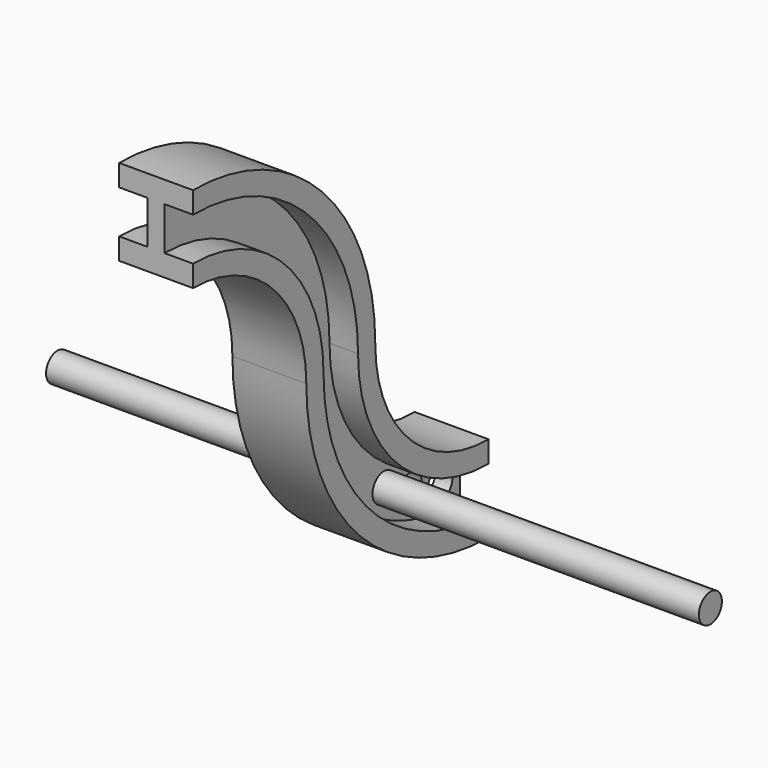
from build123d import *

# Parameters (mm, degrees)
F3_R     = 29.6946462183
F4_DEPTH = 673.1
F5_R     = 31.777125294
F5_R_2   = 32.6810684337
F6_DEPTH = 673.101


# Not quite as in the source:
# - a feature of the source that left no trace in its solid (it failed there, or was rolled back) is left out


with BuildPart() as f2:
    # F2: sweep along a path in F1
    with BuildLine(Plane.YZ) as f2_path:
        ThreePointArc((0, 0), (269.4076836321, -111.5923163679), (381, -381))
        ThreePointArc((381, -381), (492.5923163679, -650.4076836321), (762, -762))
    # F0 (on Front) → F2 (sweep)
    with BuildSketch(Plane.XZ):
        Polygon((76.2, 88.9), (0, 88.9), (-76.2, 88.9), (-76.2, 44.45), (-17.3748321831, 44.45), (-17.3748321831, 0), (-17.3748321831, -44.45), (-76.2, -44.45), (-76.2, -88.9), (0, -88.9), (76.2, -88.9), (76.2, -44.45), (17.3748321831, -44.45), (17.3748321831, 0), (17.3748321831, 44.45), (76.2, 44.45), align=None)
    sweep(path=f2_path.line)

    # F3 (on face) → F4 (join, symmetric)
    with BuildSketch(Plane.YZ.offset(17.3748321831)):
        with Locations((565.865278244, -699.9046206474)):
            Circle(F3_R)
    extrude(amount=F4_DEPTH, both=True)

    # F5 (on face) → F6 (cut, through all)
    with BuildSketch(Plane.YZ.offset(17.3748321831)):
        with Locations((631.9480538368, -732.2566509247)):
            Circle(F5_R)
        with Locations((709.6602916718, -753.0537247658)):
            Circle(F5_R_2)
    extrude(amount=-F6_DEPTH, mode=Mode.SUBTRACT)


solid = f2.part
